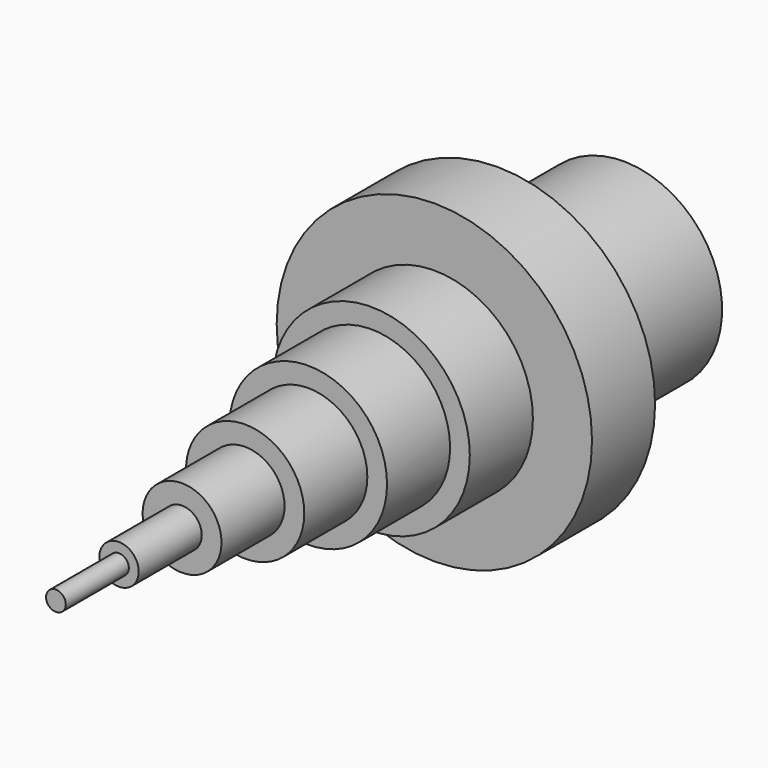
from build123d import *

# Parameters (mm, degrees)
F0_R      = 40
F1_DEPTH  = 20
F2_R      = 25
F3_DEPTH  = 20
F4_R      = 20
F5_DEPTH  = 20
F6_R      = 15
F7_DEPTH  = 20
F8_R      = 10
F9_DEPTH  = 20
F10_R     = 5
F11_DEPTH = 20
F12_R     = 2.5
F13_DEPTH = 20
F14_R     = 25
F15_DEPTH = 40
F16_R     = 20
F17_DEPTH = 40


# Not quite as in the source:
# - a feature names something its author has since deleted; it is built from what else it names


with BuildPart() as f1:
    # F0 (on Front) → F1 (new body)
    with BuildSketch(Plane.XZ):
        Circle(F0_R)
    extrude(amount=F1_DEPTH)

    # F2 (on face) → F3 (join)
    with BuildSketch(Plane.XZ.offset(20)):
        Circle(F2_R)
    extrude(amount=F3_DEPTH)

    # F4 (on face) → F5 (join)
    with BuildSketch(Plane.XZ.offset(40)):
        Circle(F4_R)
    extrude(amount=F5_DEPTH)

    # F6 (on face) → F7 (join)
    with BuildSketch(Plane.XZ.offset(60)):
        Circle(F6_R)
    extrude(amount=F7_DEPTH)

    # F8 (on face) → F9 (join)
    with BuildSketch(Plane.XZ.offset(80)):
        Circle(F8_R)
    extrude(amount=F9_DEPTH)

    # F10 (on face) → F11 (join)
    with BuildSketch(Plane.XZ.offset(100)):
        Circle(F10_R)
    extrude(amount=F11_DEPTH)

    # F12 (on face) → F13 (join)
    with BuildSketch(Plane.XZ.offset(120)):
        Circle(F12_R)
    extrude(amount=F13_DEPTH)

    # F14 (on face) → F15 (join)
    with BuildSketch(Plane(origin=(0, 0, 0), x_dir=(-1, 0, 0), z_dir=(0, 1, 0))):
        Circle(F14_R)
    extrude(amount=F15_DEPTH)

    # F16 (on face) → F17 (cut)
    with BuildSketch(Plane(origin=(0, 40, 0), x_dir=(-1, 0, 0), z_dir=(0, 1, 0))):
        Circle(F16_R)
    extrude(amount=-F17_DEPTH, mode=Mode.SUBTRACT)


solid = f1.part
